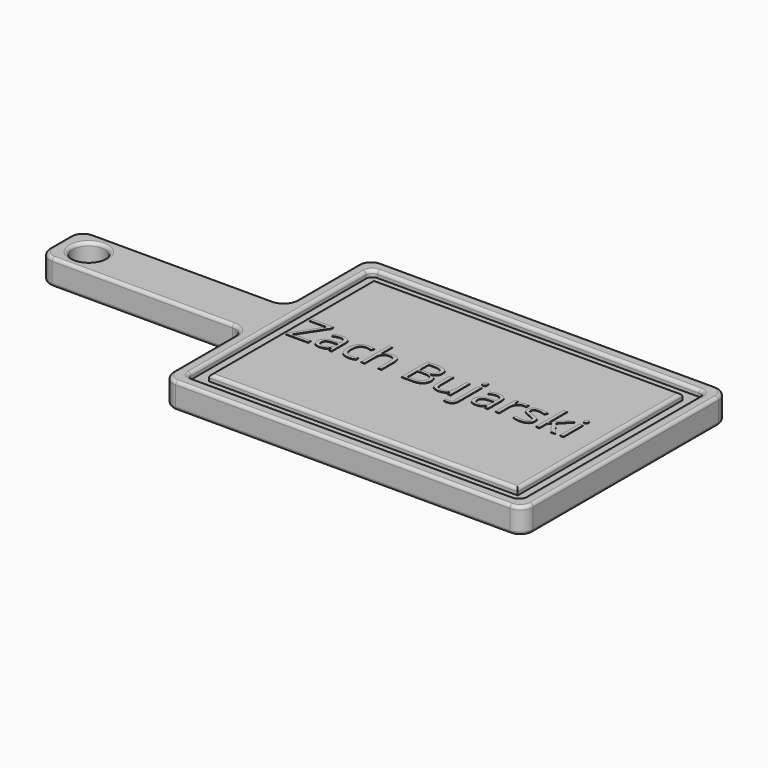
from build123d import *

# Parameters (mm, degrees)
F0_W         = 203.2
F0_H         = 50.8
F1_DEPTH     = 25.4
F2_R         = 15.875
F3_DEPTH     = 25.4
F5_DEPTH     = 6.35
F6_R         = 6.35
F7_R         = 12.7
F8_R         = 3.175
F9_TEXT_SIZE = 45.0849679794
F10_DEPTH    = 0.508


# Not quite as in the source:
# - Text() gives the source's letters only with a copy of the font that has no kerning and outlines rounded to 1/6400 em; it was checked with that copy


with BuildPart() as f1:
    # F0 (on Top) → F1 (new body)
    with BuildSketch(Plane.XY):
        Polygon((0, 101.6), (0, 0), (355.6, 0), (355.6, 254), (0, 254), (0, 152.4), align=None)
        with Locations((-101.6, 127)):
            Rectangle(F0_W, F0_H)
    extrude(amount=F1_DEPTH)

    # F2 (on face) → F3 (cut)
    with BuildSketch(Plane.XY.offset(25.4)):
        with Locations((-174.625, 126.873)):
            Circle(F2_R)
    extrude(amount=-F3_DEPTH, mode=Mode.SUBTRACT)

    # F4 (on face) → F5 (cut)
    with BuildSketch(Plane.XY.offset(25.4)):
        Polygon((12.7, 101.6), (12.7, 12.7), (342.9, 12.7), (342.9, 241.3), (12.7, 241.3), (12.7, 152.4), align=None)
        Polygon((25.4, 101.6), (25.4, 152.4), (25.4, 228.6), (330.2, 228.6), (330.2, 25.4), (25.4, 25.4), align=None, mode=Mode.SUBTRACT)
    extrude(amount=-F5_DEPTH, mode=Mode.SUBTRACT)

    # F6
    f6_edges = [f1.edges().sort_by_distance(p)[0] for p in [
        (12.7, 241.3, 22.225),
        (342.9, 241.3, 22.225),
        (342.9, 12.7, 22.225),
        (12.7, 12.7, 22.225),
    ]]
    fillet(f6_edges, radius=F6_R)

    # F7
    f7_edges = [f1.edges().sort_by_distance(p)[0] for p in [
        (0, 0, 12.7),
        (-203.2, 101.6, 12.7),
        (-203.2, 152.4, 12.7),
        (0, 254, 12.7),
        (355.6, 0, 12.7),
        (355.6, 254, 12.7),
        (0, 101.6, 12.7),
        (0, 152.4, 12.7),
    ]]
    fillet(f7_edges, radius=F7_R)

    # F8
    f8_edges = [f1.edges().sort_by_distance(p)[0] for p in [
        (177.8, 228.6, 25.4),
        (330.2, 127, 25.4),
        (177.8, 25.4, 25.4),
        (25.4, 127, 25.4),
        (0, 50.8, 25.4),
        (-3.719744, 97.880256, 25.4),
        (3.719744, 3.719744, 25.4),
        (-101.6, 101.6, 25.4),
        (177.8, 0, 25.4),
        (-199.480256, 105.319744, 25.4),
        (351.880256, 3.719744, 25.4),
        (-203.2, 127, 25.4),
        (355.6, 127, 25.4),
        (-199.480256, 148.680256, 25.4),
        (351.880256, 250.280256, 25.4),
        (-101.6, 152.4, 25.4),
        (177.8, 254, 25.4),
        (-3.719744, 156.119744, 25.4),
        (3.719744, 250.280256, 25.4),
        (0, 203.2, 25.4),
        (177.8, 12.7, 25.4),
        (14.559872, 14.559872, 25.4),
        (341.040128, 14.559872, 25.4),
        (12.7, 127, 25.4),
        (342.9, 127, 25.4),
        (14.559872, 239.440128, 25.4),
        (341.040128, 239.440128, 25.4),
        (177.8, 241.3, 25.4),
        (-190.5, 126.873, 25.4),
        (0, 50.8, 0),
        (-3.719744, 97.880256, 0),
        (3.719744, 3.719744, 0),
        (-101.6, 101.6, 0),
        (177.8, 0, 0),
        (-199.480256, 105.319744, 0),
        (351.880256, 3.719744, 0),
        (-203.2, 127, 0),
        (355.6, 127, 0),
        (-199.480256, 148.680256, 0),
        (351.880256, 250.280256, 0),
        (-101.6, 152.4, 0),
        (177.8, 254, 0),
        (-3.719744, 156.119744, 0),
        (3.719744, 250.280256, 0),
        (0, 203.2, 0),
        (-190.5, 126.873, 0),
    ]]
    fillet(f8_edges, radius=F8_R)

    # F9 (on face) → F10 (join)
    with BuildSketch(Plane.XY.offset(25.4)):
        with Locations((28.575, 113.7947589159)):
            Text('Zach Bujarski', F9_TEXT_SIZE, font='Open Sans', text_align=(TextAlign.LEFT, TextAlign.BOTTOM))
    extrude(amount=F10_DEPTH)


solid = f1.part
